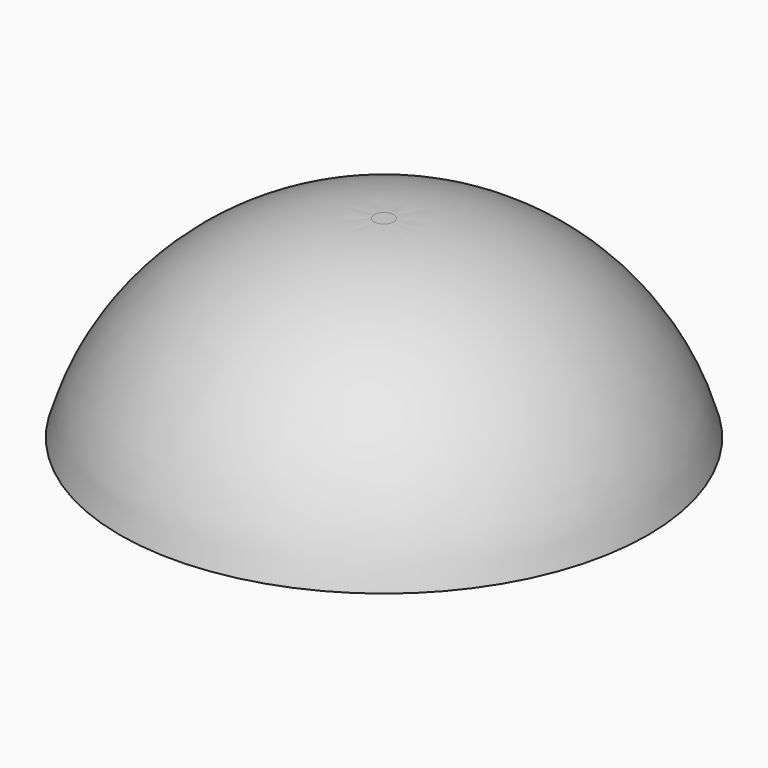
from build123d import *

# Parameters (mm, degrees)
F0_R     = 34.7763099746
F1_DEPTH = 25.4


# Not quite as in the source:
# - a fillet or chamfer that OpenCascade refuses, or shapes differently, is made with other operations: its cross-section is extruded or revolved along the edge and cut away or added


with BuildPart() as f1:
    # F0 (on Top) → F1 (new body)
    with BuildSketch(Plane.XY):
        Circle(F0_R)
    extrude(amount=F1_DEPTH)

    # F2: fillet of radius 34.7726 on 1 edges, made by hand

    # F2_s1 → F2_t2 (revolve, cut)
    with BuildSketch(Plane.XZ):
        with BuildLine():
            ThreePointArc((34.7763099746, 0), (22.3052369198, 18.331581828), (1.2906700673, 25.4))
            Line((1.2906700673, 25.4), (34.7763099746, 25.4))
            Line((34.7763099746, 25.4), (34.7763099746, 0))
        make_face()
    revolve(axis=Axis((0, 0, 25.4), (0, 0, 1)), mode=Mode.SUBTRACT)


solid = f1.part
